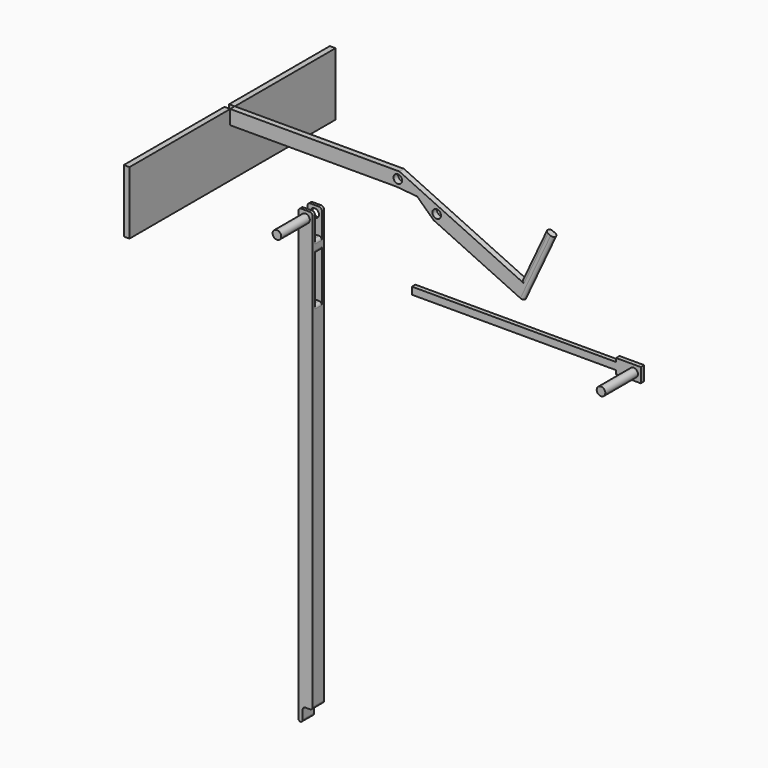
from build123d import *

# Parameters (mm, degrees)
F0_R        = 1.5
F1_DEPTH    = 0.75
F0_W        = 5
F0_H        = 12.5
F0_H_2      = 16
F2_DEPTH    = 2.5
F3_DEPTH    = 1
F4_DEPTH    = 45
F5_W        = 3
F5_H        = 9
F5_H_2      = 16
F6_DEPTH    = 118.2633225451
F7_T1_DEPTH = 5
F7_T3_DEPTH = 6
F7_T5_DEPTH = 6
F7_T7_DEPTH = 10
F7_T9_DEPTH = 3
F7_2_F1_R   = 1
F7_2_F2_R   = 0.9999
F7_2_F3_R   = 1
F7_2_F4_R   = 0.9999
F9_W        = 2
F9_H        = 5
F10_DEPTH   = 25
F11_DEPTH   = 15


# Not quite as in the source:
# - a fillet or chamfer that OpenCascade refuses, or shapes differently, is made with other operations: its cross-section is extruded or revolved along the edge and cut away or added
# - two fillets or chamfers of one size are made in one step
# - a fillet or chamfer is up to 0.001 mm smaller than in the source, because OpenCascade refuses the exact size


with BuildPart() as f1:
    # F0 (on Front) → F1 (new body, symmetric)
    with BuildSketch(Plane.XZ):
        Polygon((-6.2327417545, 42.8849308193), (-77.6071324944, 42.8849308193), (-77.6071324944, 40.3849308193), (-6.2327417545, 40.3849308193), (-6.2327417545, 41.6349308193), align=None)
        Polygon((2.3928675056, 44.1349308193), (-6.2327417545, 44.1349308193), (-6.2327417545, 42.8849308193), (-6.2327417545, 41.6349308193), (-6.2327417545, 40.3849308193), (-6.2327417545, 39.1349308193), (2.3928675056, 39.1349308193), align=None)
        with Locations((-0.1071324944, 41.6349308193)):
            Circle(F0_R, mode=Mode.SUBTRACT)
    extrude(amount=F1_DEPTH, both=True)


with BuildPart() as f2:
    # F0 (on Front) → F2 (new body, symmetric)
    with BuildSketch(Plane.XZ):
        with Locations((-113.3694550395, 49.191441834)):
            Rectangle(F0_W, F0_H)
        with Locations((-113.3694550395, 52.941441834)):
            Circle(F0_R, mode=Mode.SUBTRACT)
        Polygon((-110.8694550395, 26.941441834), (-115.8694550395, 26.941441834), (-115.8694550395, -102.558558166), (-114.3694550395, -102.558558166), (-114.3694550395, -97.558558166), (-112.3694550395, -97.558558166), (-110.8694550395, -97.558558166), align=None)
        with Locations((-113.3694550395, 34.941441834)):
            Rectangle(F0_W, F0_H_2)
    extrude(amount=F2_DEPTH, both=True)

    # F5 (on face) → F6 (cut, through all)
    with BuildSketch(Plane(origin=(-115.8694550395, 0, 0), x_dir=(0, -1, 0), z_dir=(-1, 0, 0))):
        with Locations((0, 50.941441834)):
            Rectangle(F5_W, F5_H)
        with Locations((0, 34.441441834)):
            Rectangle(F5_W, F5_H_2)
    extrude(amount=-F6_DEPTH, mode=Mode.SUBTRACT)

    # F7: fillet of radius 1 on 14 edges, made by hand

    # F7_s2 → F7_t1 (join)
    with BuildSketch(Plane.XZ.offset(-2.5)):
        with BuildLine():
            ThreePointArc((-113.3694550395, -97.558558166), (-114.0765618207, -97.8514513848), (-114.3694550395, -98.558558166))
            Line((-114.3694550395, -98.558558166), (-114.3694550395, -97.558558166))
            Line((-114.3694550395, -97.558558166), (-113.3694550395, -97.558558166))
        make_face()
    extrude(amount=F7_T1_DEPTH)

    # F7_s4 → F7_t3 (cut)
    with BuildSketch(Plane.XZ.offset(-1)):
        with BuildLine():
            ThreePointArc((-110.8694550395, 54.441441834), (-111.1623482583, 55.1485486152), (-111.8694550395, 55.441441834))
            Line((-111.8694550395, 55.441441834), (-110.8694550395, 55.441441834))
            Line((-110.8694550395, 55.441441834), (-110.8694550395, 54.441441834))
        make_face()
        with BuildLine():
            ThreePointArc((-115.8694550395, 54.441441834), (-115.5765618207, 55.1485486152), (-114.8694550395, 55.441441834))
            Line((-114.8694550395, 55.441441834), (-115.8694550395, 55.441441834))
            Line((-115.8694550395, 55.441441834), (-115.8694550395, 54.441441834))
        make_face()
    extrude(amount=F7_T3_DEPTH, mode=Mode.SUBTRACT)

    # F7_s6 → F7_t5 (cut)
    with BuildSketch(Plane.XZ.offset(-5)):
        with BuildLine():
            ThreePointArc((-111.8694550395, 55.441441834), (-111.1623482583, 55.1485486152), (-110.8694550395, 54.441441834))
            Line((-110.8694550395, 54.441441834), (-110.8694550395, 55.441441834))
            Line((-110.8694550395, 55.441441834), (-111.8694550395, 55.441441834))
        make_face()
        with BuildLine():
            ThreePointArc((-114.8694550395, 55.441441834), (-115.5765618207, 55.1485486152), (-115.8694550395, 54.441441834))
            Line((-115.8694550395, 54.441441834), (-115.8694550395, 55.441441834))
            Line((-115.8694550395, 55.441441834), (-114.8694550395, 55.441441834))
        make_face()
    extrude(amount=F7_T5_DEPTH, mode=Mode.SUBTRACT)

    # F7_s8 → F7_t7 (cut)
    with BuildSketch(Plane.XZ.offset(-5)):
        with BuildLine():
            ThreePointArc((-115.3694550395, -102.558558166), (-114.6623482583, -102.2656649472), (-114.3694550395, -101.558558166))
            Line((-114.3694550395, -101.558558166), (-114.3694550395, -102.558558166))
            Line((-114.3694550395, -102.558558166), (-115.3694550395, -102.558558166))
        make_face()
        with BuildLine():
            ThreePointArc((-115.8694550395, -101.558558166), (-115.5765618207, -102.2656649472), (-114.8694550395, -102.558558166))
            Line((-114.8694550395, -102.558558166), (-115.8694550395, -102.558558166))
            Line((-115.8694550395, -102.558558166), (-115.8694550395, -101.558558166))
        make_face()
        with BuildLine():
            ThreePointArc((-110.8694550395, -96.558558166), (-111.1623482583, -97.2656649472), (-111.8694550395, -97.558558166))
            Line((-111.8694550395, -97.558558166), (-110.8694550395, -97.558558166))
            Line((-110.8694550395, -97.558558166), (-110.8694550395, -96.558558166))
        make_face()
    extrude(amount=F7_T7_DEPTH, mode=Mode.SUBTRACT)

    # F7_s10 → F7_t9 (cut)
    with BuildSketch(Plane.XZ.offset(-1.5)):
        with BuildLine():
            ThreePointArc((-110.8694550395, 43.441441834), (-111.1623482583, 42.7343350528), (-111.8694550395, 42.441441834))
            Line((-111.8694550395, 42.441441834), (-110.8694550395, 42.441441834))
            Line((-110.8694550395, 42.441441834), (-110.8694550395, 43.441441834))
        make_face()
        with BuildLine():
            ThreePointArc((-110.8694550395, 25.441441834), (-111.1623482583, 26.1485486152), (-111.8694550395, 26.441441834))
            Line((-111.8694550395, 26.441441834), (-110.8694550395, 26.441441834))
            Line((-110.8694550395, 26.441441834), (-110.8694550395, 25.441441834))
        make_face()
        with BuildLine():
            ThreePointArc((-115.8694550395, 43.441441834), (-115.5765618207, 42.7343350528), (-114.8694550395, 42.441441834))
            Line((-114.8694550395, 42.441441834), (-115.8694550395, 42.441441834))
            Line((-115.8694550395, 42.441441834), (-115.8694550395, 43.441441834))
        make_face()
        with BuildLine():
            ThreePointArc((-115.8694550395, 25.441441834), (-115.5765618207, 26.1485486152), (-114.8694550395, 26.441441834))
            Line((-114.8694550395, 26.441441834), (-115.8694550395, 26.441441834))
            Line((-115.8694550395, 26.441441834), (-115.8694550395, 25.441441834))
        make_face()
        with BuildLine():
            ThreePointArc((-115.8694550395, 45.441441834), (-115.5765618207, 46.1485486152), (-114.8694550395, 46.441441834))
            Line((-114.8694550395, 46.441441834), (-115.8694550395, 46.441441834))
            Line((-115.8694550395, 46.441441834), (-115.8694550395, 45.441441834))
        make_face()
        with BuildLine():
            ThreePointArc((-110.8694550395, 45.441441834), (-111.1623482583, 46.1485486152), (-111.8694550395, 46.441441834))
            Line((-111.8694550395, 46.441441834), (-110.8694550395, 46.441441834))
            Line((-110.8694550395, 46.441441834), (-110.8694550395, 45.441441834))
        make_face()
    extrude(amount=F7_T9_DEPTH, mode=Mode.SUBTRACT)


with BuildPart() as f3:
    # F0 (on Front) → F3 (new body, symmetric)
    with BuildSketch(Plane.XZ):
        Polygon((-81.7702353249, 77.0455077887), (-140.8787086381, 77.0455077887), (-140.8787086381, 72.0455077887), (-82.8787086381, 72.0455077887), (-75.5537198958, 71.3882542396), (-69.7864008303, 65.940464395), (-38.5679372817, 51.3830557664), (-36.454845973, 55.9145947016), (-39.1737693341, 57.1824494868), align=None)
        with Locations((-82.3244719815, 74.5455077887)):
            Circle(F0_R, mode=Mode.SUBTRACT)
        with Locations((-68.7298551759, 68.2062338625)):
            Circle(F0_R, mode=Mode.SUBTRACT)
        Polygon((-30.7214040993, 75.3086052276), (-39.1737693341, 57.1824494868), (-36.454845973, 55.9145947016), (-28.0024807382, 74.0407504424), align=None)
    extrude(amount=F3_DEPTH, both=True)

    # F7#2: fillet of radius 1 on 4 edges, made by hand

    # F7_2_f1
    f7_2_f1_edges = [f3.edges().sort_by_distance(p)[0] for p in [
        (-34.9475867167, 1, 66.2455273572),
    ]]
    fillet(f7_2_f1_edges, radius=F7_2_F1_R)

    # F7_2_f2 (radius 1 in the source; OpenCascade refuses exactly that, so slightly less here)
    f7_2_f2_edges = [f3.edges().sort_by_distance(p)[0] for p in [
        (-34.9475867167, -1, 66.2455273572),
    ]]
    fillet(f7_2_f2_edges, radius=F7_2_F2_R)

    # F7_2_f3
    f7_2_f3_edges = [f3.edges().sort_by_distance(p)[0] for p in [
        (-33.28520901, 1, 62.7119031044),
    ]]
    fillet(f7_2_f3_edges, radius=F7_2_F3_R)

    # F7_2_f4 (radius 1 in the source; OpenCascade refuses exactly that, so slightly less here)
    f7_2_f4_edges = [f3.edges().sort_by_distance(p)[0] for p in [
        (-33.28520901, -1, 62.7119031044),
    ]]
    fillet(f7_2_f4_edges, radius=F7_2_F4_R)


with BuildPart() as f4:
    # F0 (on Front) → F4 (new body, symmetric)
    with BuildSketch(Plane.XZ):
        Polygon((-140.8787086381, 77.0455077887), (-142.8787086381, 77.0455077887), (-142.8787086381, 55.0455077887), (-140.8787086381, 55.0455077887), (-140.8787086381, 72.0455077887), align=None)
    extrude(amount=F4_DEPTH, both=True)

    # F9 (on face) → F10 (cut)
    with BuildSketch(Plane(origin=(-142.8787086381, 0, 0), x_dir=(0, -1, 0), z_dir=(-1, 0, 0))):
        with Locations((0, 74.5455077887)):
            Rectangle(F9_W, F9_H)
    extrude(amount=-F10_DEPTH, mode=Mode.SUBTRACT)


with BuildPart() as f11:
    # F0 (on Front) → F11 (new body)
    with BuildSketch(Plane.XZ):
        with Locations((-113.3694550395, 52.941441834)):
            Circle(F0_R)
    extrude(amount=F11_DEPTH)


with BuildPart() as f11b:
    # F0 (on Front) → F11, piece 2 (new body)
    with BuildSketch(Plane.XZ):
        with Locations((-0.1071324944, 41.6349308193)):
            Circle(F0_R)
    extrude(amount=F11_DEPTH)


solid = Compound([f1.part, f2.part, f3.part, f4.part, f11.part, f11b.part])
